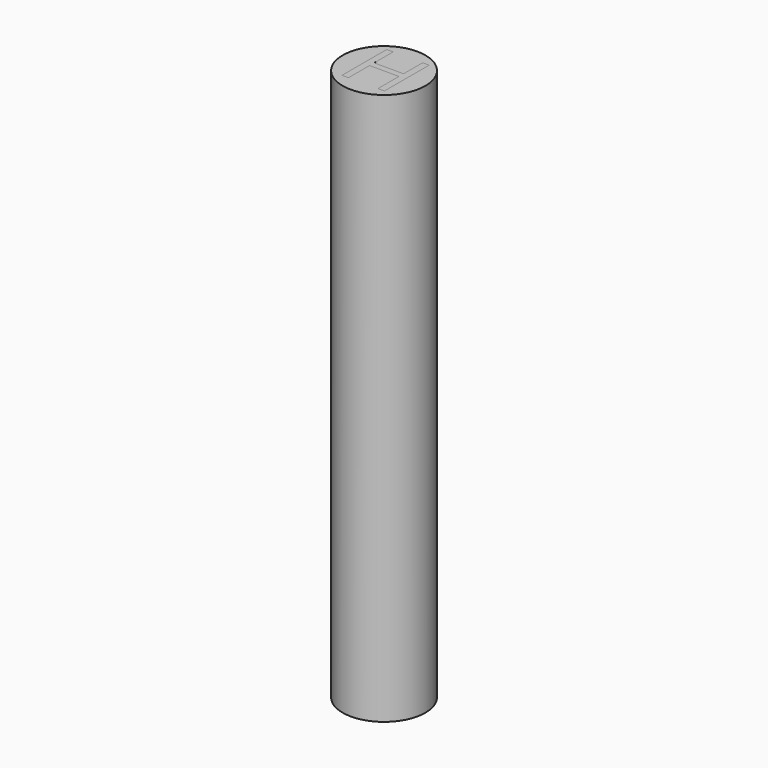
from build123d import *

# Parameters (mm, degrees)
F0_R         = 3.81
F1_DEPTH     = 25.4
F2_TEXT_SIZE = 7.2056737589
F3_DEPTH     = 0.000254
F4_TEXT_SIZE = 7.2056737589
F5_DEPTH     = 0.000254


# Not quite as in the source:
# - Text() gives the source's letters only with a copy of the font that has no kerning and outlines rounded to 1/6400 em; it was checked with that copy


with BuildPart() as f1:
    # F0 (on Top) → F1 (new body, symmetric)
    with BuildSketch(Plane.XY):
        Circle(F0_R)
    extrude(amount=F1_DEPTH, both=True)

    # F2 (on face) → F3 (join)
    with BuildSketch(Plane.XY.offset(25.4)):
        with Locations((-2.6052925026, -2.4675240703)):
            Text('H', F2_TEXT_SIZE, font='Open Sans', text_align=(TextAlign.LEFT, TextAlign.BOTTOM))
    extrude(amount=F3_DEPTH)

    # F4 (on face) → F5 (join)
    with BuildSketch(Plane(origin=(0, 0, -25.4), x_dir=(1, 0, 0), z_dir=(0, 0, -1))):
        with Locations((-2.5673190304, -2.553691728)):
            Text('H', F4_TEXT_SIZE, font='Open Sans', text_align=(TextAlign.LEFT, TextAlign.BOTTOM))
    extrude(amount=F5_DEPTH)


solid = f1.part
